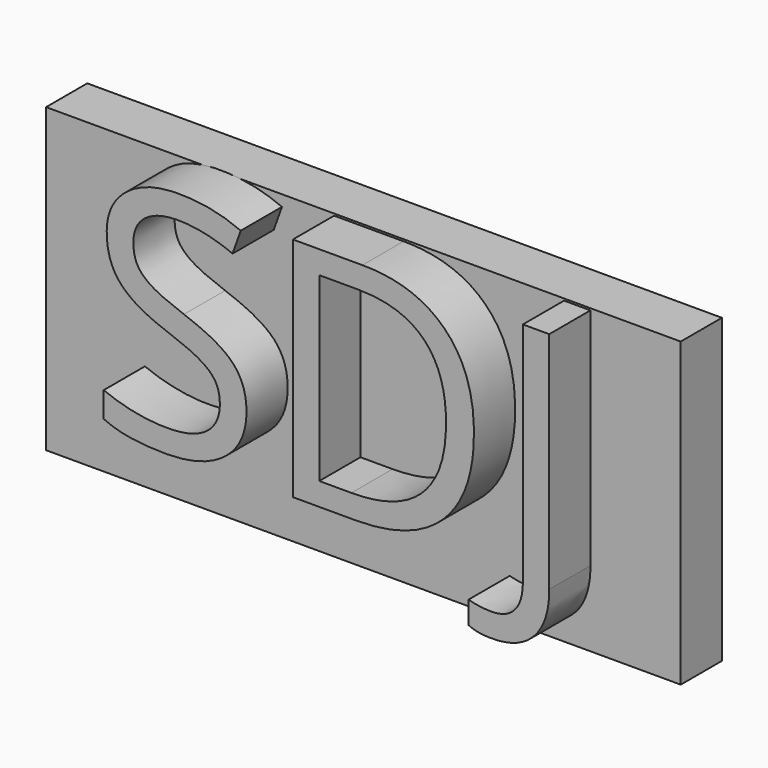
from build123d import *

# Parameters (mm, degrees)
F0_W         = 93.9287915826
F0_H         = 44.7060503066
F1_DEPTH     = 7.62
F2_TEXT_SIZE = 47.0284825294
F3_DEPTH     = 7.62


# Not quite as in the source:
# - Text() gives the source's letters only with a copy of the font that has no kerning and outlines rounded to 1/6400 em; it was checked with that copy


with BuildPart() as f1:
    # F0 (on Front) → F1 (new body)
    with BuildSketch(Plane.XZ):
        with Locations((46.9643957913, 22.3530251533)):
            Rectangle(F0_W, F0_H)
    extrude(amount=F1_DEPTH)

    # F2 (on face) → F3 (join)
    with BuildSketch(Plane.XZ.offset(7.62)):
        with Locations((12.1967503348, 10.8455428854)):
            Text('SDJ', F2_TEXT_SIZE, font='Open Sans', text_align=(TextAlign.LEFT, TextAlign.BOTTOM))
    extrude(amount=F3_DEPTH)


solid = f1.part
